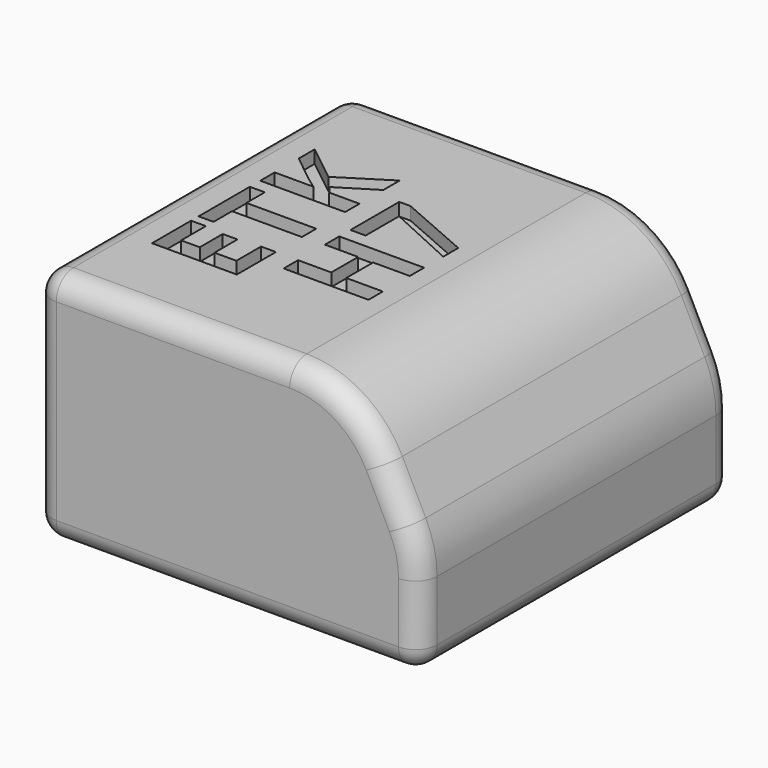
from build123d import *

# Parameters (mm, degrees)
F1_DEPTH     = 91.5
F2_R         = 5
F3_TEXT_SIZE = 27.7777777778
F4_TEXT_SIZE = 27.7777777778
F5_DEPTH     = 3


# Not quite as in the source:
# - Text() gives the source's letters only with a copy of the font that has no kerning and outlines rounded to 1/6400 em; it was checked with that copy


with BuildPart() as f1:
    # F0 (on Front) → F1 (new body)
    with BuildSketch(Plane.XZ):
        with BuildLine():
            Line((0, 55), (0, 0))
            Line((0, 0), (90, 0))
            Line((90, 0), (90, 19.0983005625))
            ThreePointArc((90, 19.0983005625), (89.3312247367, 24.8421235762), (87.360679775, 30.27864045))
            Line((87.360679775, 30.27864045), (81.9098300563, 41.1803398875))
            ThreePointArc((81.9098300563, 41.1803398875), (72.6924280842, 51.2662702088), (59.5491502813, 55))
            Line((59.5491502813, 55), (0, 55))
        make_face()
    extrude(amount=F1_DEPTH)

    # F2
    f2_edges = [f1.edges().sort_by_distance(p)[0] for p in [
        (29.774575, -91.5, 55),
        (0, -91.5, 27.5),
        (45, -91.5, 0),
        (29.774575, 0, 55),
        (45, 0, 0),
        (0, 0, 27.5),
        (0, -45.75, 0),
        (0, -45.75, 55),
        (90, -45.75, 0),
    ]]
    fillet(f2_edges, radius=F2_R)

    # F3 (on face) + F4 (on face) → F5 (cut)
    with BuildSketch(Plane.XY.offset(55)):
        with Locations(Location((30, -72.5), (0, 0, 90))):
            Text('ETK', F3_TEXT_SIZE, font='Open Sans', font_style=FontStyle.BOLD, text_align=(TextAlign.LEFT, TextAlign.BOTTOM))
    with BuildSketch(Plane.XY.offset(55)):
        with Locations(Location((55, -65.2821180556), (0, 0, 90))):
            Text('H7', F4_TEXT_SIZE, font='Open Sans', font_style=FontStyle.BOLD, text_align=(TextAlign.LEFT, TextAlign.BOTTOM))
    extrude(amount=-F5_DEPTH, mode=Mode.SUBTRACT)


solid = f1.part
